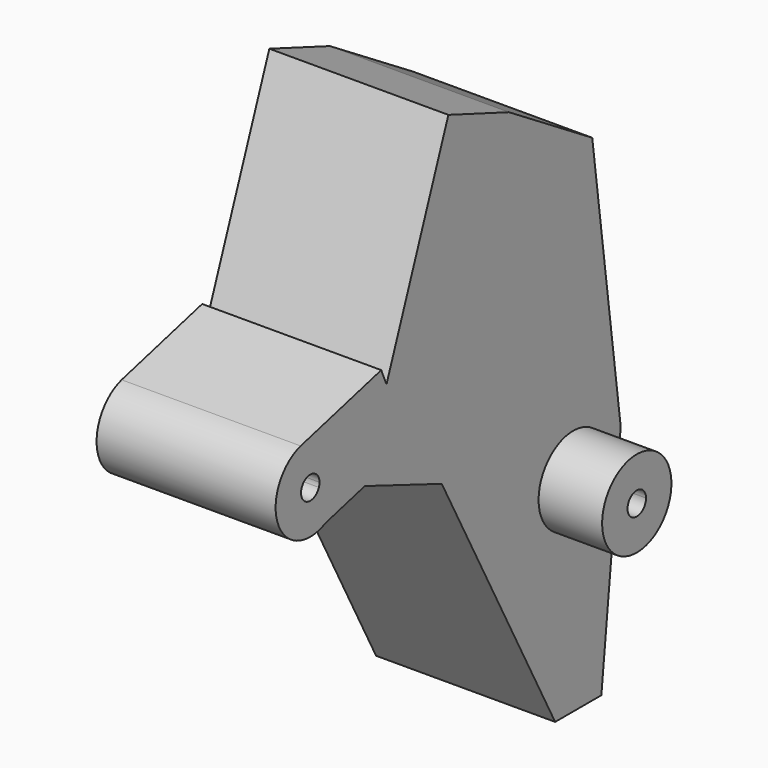
from build123d import *

# Parameters (mm, degrees)
F3_DEPTH      = 15
F3_DEPTH_BACK = 16
F4_DEPTH      = 26
F4_DEPTH_BACK = 26
F6_DEPTH      = 25
F6_DEPTH_BACK = 25


# Not quite as in the source:
# - a feature names something its author has since deleted; it is built from what else it names


with BuildPart() as f3:
    # F0 (on Right) → F3 (new body, two sides)
    with BuildSketch(Plane.YZ) as f3_sk:
        Polygon((42.99440903, 39.7499332097), (24.4999610724, -9.4537481835), (28.4550828122, -10.9799026477), (53, -57.2503693402), (63, -57.2503693402), (67.1839944136, -18.0194567546), (61.0229901087, 28.5260152414), align=None)
        with BuildLine():
            ThreePointArc((64.4101656244, -21.9598052953), (55.5369643161, -29.3330215655), (49.9130141132, -19.2598292344))
            ThreePointArc((49.9130141132, -19.2598292344), (58.2833669326, -14.5865890251), (64.4101656244, -21.9598052953))
        make_face(mode=Mode.SUBTRACT)
        with BuildLine():
            Line((3.3187451802, -6.7257661592), (11.7920777761, -4.5501841217))
            Line((11.7920777761, -4.5501841217), (18.186862473, -7.0177261735))
            Line((18.186862473, -7.0177261735), (24.4999610724, -9.4537481835))
            Line((24.4999610724, -9.4537481835), (42.99440903, 39.7499332097))
            Line((42.99440903, 39.7499332097), (28.0174564582, 45.3793995842))
            Line((28.0174564582, 45.3793995842), (15.3511571156, 11.6812562976))
            Line((15.3511571156, 11.6812562976), (-2.0833397847, 7.2048383286))
            ThreePointArc((-2.0833397847, 7.2048383286), (-6.9926384128, -2.7116430495), (3.3187451802, -6.7257661592))
        make_face()
        with BuildLine():
            ThreePointArc((2, 0), (1.9661910054, -0.3661870155), (1.8659070697, -0.7199936162))
            ThreePointArc((1.8659070697, -0.7199936162), (-1.9661910054, 0.3661870155), (2, 0))
        make_face(mode=Mode.SUBTRACT)
    extrude(amount=F3_DEPTH)
    extrude(f3_sk.sketch, amount=-F3_DEPTH_BACK)

    # F0 (on Right) → F4 (join, two sides)
    with BuildSketch(Plane.YZ) as f4_sk:
        with BuildLine():
            ThreePointArc((64.4101656244, -21.9598052953), (58.2833669326, -14.5865890251), (49.9130141132, -19.2598292344))
            ThreePointArc((49.9130141132, -19.2598292344), (55.5369643161, -29.3330215655), (64.4101656244, -21.9598052953))
        make_face()
        with BuildLine():
            ThreePointArc((58.9101656244, -21.9598052953), (56.5439786088, -23.9259963007), (55.0442585547, -21.2398116791))
            ThreePointArc((55.0442585547, -21.2398116791), (57.2763526399, -19.9936142899), (58.9101656244, -21.9598052953))
        make_face(mode=Mode.SUBTRACT)
    extrude(amount=F4_DEPTH)
    extrude(f4_sk.sketch, amount=-F4_DEPTH_BACK)

    # F5 (on Right) → F6 (cut, two sides)
    with BuildSketch(Plane.YZ) as f6_sk:
        Polygon((16.4947576102, 9.0393807374), (29.8895755297, 44.6757162874), (28.0174564582, 45.3793995842), (15.3511571156, 11.6812562976), align=None)
    extrude(amount=-F6_DEPTH, mode=Mode.SUBTRACT)
    extrude(f6_sk.sketch, amount=F6_DEPTH_BACK, mode=Mode.SUBTRACT)


solid = f3.part
